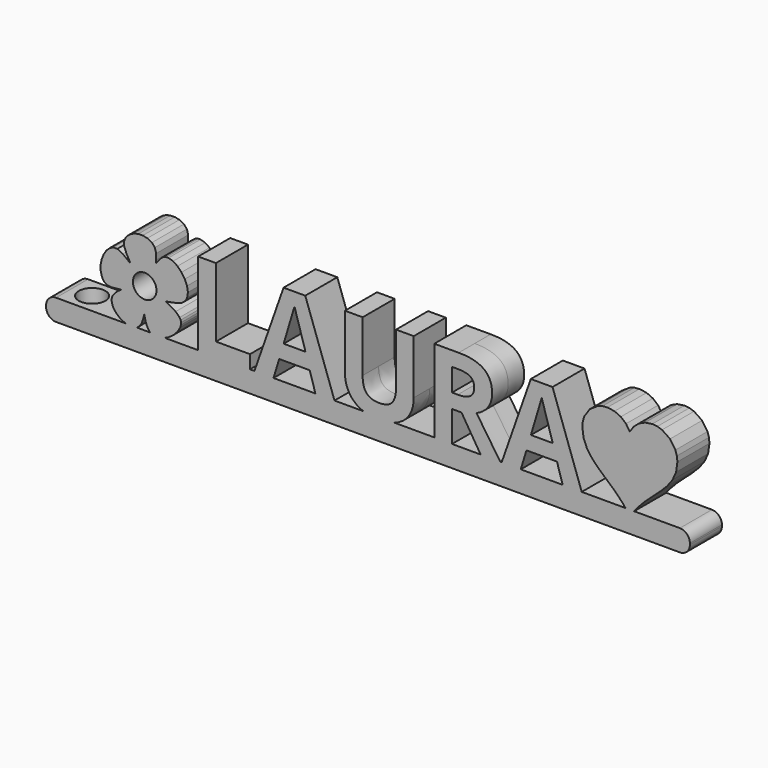
from build123d import *

# Parameters (mm, degrees)
F0_R         = 1.7660260944
F0_TEXT_SIZE = 17.5961359837
F1_DEPTH     = 3
F2_W         = 89
F2_H         = 6
F3_DEPTH     = 0.2
F4_DEPTH     = 3
F5_W         = 6
F5_H         = 3.2
F6_DEPTH     = 7.5
F7_R         = 1.5
F8_R         = 2
F9_DEPTH     = 4
F10_R        = 1.5


# Not quite as in the source:
# - Text() gives the source's letters only with a copy of the font that has no kerning and outlines rounded to 1/6400 em; it was checked with that copy


with BuildPart() as f1:
    # F0 (on Front) → F1 (new body, symmetric)
    with BuildSketch(Plane.XZ):
        Polygon((-9.8962181259, -0.0299609487), (-9.3093152472, 0.0995427735), (-8.5310452338, 0.4643787281), (-7.7886221935, 1.0156229815), (-7.1753136859, 1.6703047867), (-6.7844076966, 2.345448762), (-6.6844409889, 2.697736103), (-6.6652413988, 3.0240118702), (-6.7312263226, 3.3305926174), (-6.8868132072, 3.6238062576), (-7.4844896445, 4.1953846804), (-8.4936258745, 4.789299945), (-8.9274018823, 5.0567831788), (-8.4181052429, 5.1580766137), (-7.3131137554, 5.3695361907), (-6.5480905692, 5.6521941874), (-6.0523445823, 6.043851435), (-5.7552051187, 6.5823041299), (-5.6420905942, 7.3346827833), (-5.7751165223, 8.1369112107), (-6.1089634595, 8.9328581362), (-6.5983028952, 9.6663968681), (-7.1978267956, 10.281407439), (-7.8622157172, 10.7217585729), (-8.546147975, 10.9313258196), (-8.8812811082, 10.9320270148), (-9.2043064176, 10.8539824368), (-9.6469000392, 10.5612860557), (-10.1400767255, 9.9810366231), (-10.4508130024, 9.5801644376), (-10.4068223535, 10.0271686751), (-10.3916193646, 10.9311557532), (-10.598433195, 11.6324207168), (-11.0363252865, 12.1480644274), (-11.7143548393, 12.4951945719), (-12.3982545289, 12.6383143795), (-13.0712303381, 12.6247535348), (-13.7032208938, 12.4733707309), (-14.2641853, 12.2030313855), (-14.7240621838, 11.8325941916), (-15.0528129411, 11.3809291004), (-15.2203761991, 10.8668948051), (-15.1967042361, 10.3093544817), (-14.8286469794, 9.4077545862), (-14.3529716358, 8.5454741101), (-14.2906102139, 8.4004774316), (-14.4811582303, 8.5293860258), (-15.3946726039, 9.2300894295), (-16.21802192, 9.6332437342), (-16.8030362894, 9.634121823), (-17.3568401554, 9.3699870508), (-17.8525159958, 8.8932532172), (-18.2631576982, 8.2563454299), (-18.5618432066, 7.5116797807), (-18.7216618753, 6.7116836696), (-18.7156984739, 5.9087754295), (-18.5170445979, 5.1553756349), (-18.2008868091, 4.6439944488), (-17.7512302174, 4.3560670179), (-17.1086136552, 4.2712956407), (-16.2135760559, 4.3694053341), (-15.7044514474, 4.4302814773), (-15.6696932647, 4.4000047008), (-15.7790195709, 4.3290260096), (-16.1651405309, 4.0708069691), (-16.5523139664, 3.7127982689), (-16.8671052824, 3.3322639471), (-17.0360798838, 3.0064680418), (-17.0831036318, 2.6043628391), (-17.0239245605, 2.1921008316), (-16.867618816, 1.7819255621), (-16.6232807801, 1.3860941234), (-16.3000002503, 1.0168545414), (-15.9068693162, 0.6864593752), (-15.4529754831, 0.4071521172), (-14.9474063577, 0.1911989779), (-14.4397479673, 0.0570083052), (-13.9840845603, 0.0188926715), (-13.5797273957, 0.0772799851), (-13.2259605822, 0.2326232662), (-12.9220907946, 0.485341356), (-12.6674066752, 0.8358849825), (-12.4612081239, 1.2846821047), (-12.3027905578, 1.8321743328), (-12.1879723822, 2.2557758958), (-12.1309056827, 2.0998483864), (-12.0112204133, 1.5291342486), (-11.8237778137, 0.9902805659), (-11.5954117235, 0.5466869075), (-11.3529559319, 0.2617414835), (-10.9521058183, 0.053843468), (-10.4551700276, -0.0442881949), align=None)
        with Locations((-12.1185852993, 6.0541479067)):
            Circle(F0_R, mode=Mode.SUBTRACT)
        Polygon((58.3035863837, 12.4433699982), (57.2425663837, 12.5970599982), (56.4839563837, 12.5204799982), (55.7771563837, 12.3008699982), (54.5798163837, 11.4933499982), (53.7721963837, 10.2961199982), (53.5525463837, 9.5893599982), (53.4759563837, 8.8307599982), (53.6644763837, 7.3860999982), (54.1852163837, 6.1597099982), (54.9709663837, 5.0814099982), (55.9544963837, 4.0810299982), (58.2513463837, 2.0250499982), (59.4359363837, 0.8247399982), (60.5589263837, -0.5860800018), (60.6032063837, -0.6500000018), (60.6462363837, -0.5851400018), (61.7241463837, 0.8234499982), (62.8874463837, 2.0333299982), (65.1911163837, 4.1212499982), (66.1919063837, 5.1327499982), (66.9969063837, 6.2116199982), (67.5332963837, 7.4226699982), (67.7282763837, 8.8307599982), (67.6516963837, 9.5893599982), (67.4320863837, 10.2961199982), (66.6245663837, 11.4933499982), (65.4273363837, 12.3008699982), (64.7205663837, 12.5204799982), (63.9619763837, 12.5970599982), (62.9009563837, 12.4433699982), (61.9598863837, 12.0123599982), (61.1799363837, 11.3491699982), (60.6022663837, 10.4989199982), (60.0246063837, 11.3491699982), (59.2446563837, 12.0123599982), align=None)
        with Locations((-5.6832621215, 0)):
            Text('LAURA', F0_TEXT_SIZE, font='Open Sans', font_style=FontStyle.BOLD, text_align=(TextAlign.LEFT, TextAlign.BOTTOM))
    extrude(amount=F1_DEPTH, both=True)



with BuildPart() as f3:
    # F2 (on Top) → F3 (new body)
    with BuildSketch(Plane.XY):
        with Locations((25.1, 0)):
            Rectangle(F2_W, F2_H)
    extrude(amount=F3_DEPTH)


with BuildPart() as f4:
    # F4 (new): a face of the model
    f4_faces = [f3.part.faces().sort_by_distance(p)[0] for p in [
        (25.1, 0, 0),
    ]]
    extrude(f4_faces, amount=F4_DEPTH)


with BuildPart() as f1_1:
    add(f1.part)

    add(f3.part)  # F6 merges F3

    add(f4.part)  # F6 merges F4
    # F5 (on face) → F6 (join)
    with BuildSketch(Plane(origin=(-19.4, 0, 0), x_dir=(0, -1, 0), z_dir=(-1, 0, 0))):
        with Locations((0, -1.4)):
            Rectangle(F5_W, F5_H)
    extrude(amount=F6_DEPTH)

    # F7
    f7_edges = [f1_1.edges().sort_by_distance(p)[0] for p in [
        (-26.9, 0, -3),
        (-26.9, 0, 0.2),
        (69.6, 0, -3),
    ]]
    fillet(f7_edges, radius=F7_R)

    # F8 (on face) → F9 (cut)
    with BuildSketch(Plane.XY.offset(0.2)):
        with Locations((-22.4, 0)):
            Circle(F8_R)
    extrude(amount=-F9_DEPTH, mode=Mode.SUBTRACT)

    # F10
    f10_edges = [f1_1.edges().sort_by_distance(p)[0] for p in [
        (69.6, 0, 0.2),
    ]]
    fillet(f10_edges, radius=F10_R)


solid = f1_1.part
